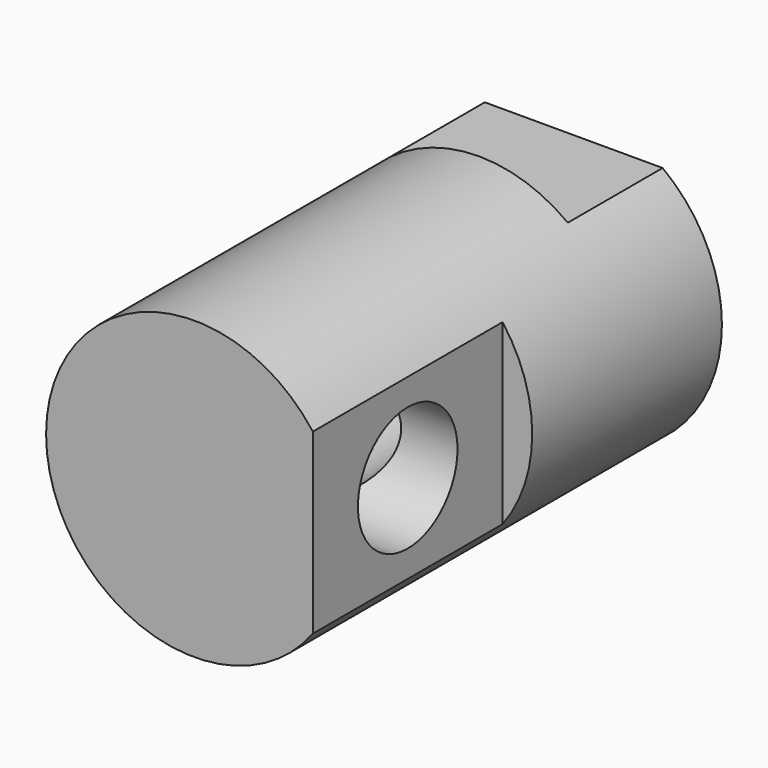
from build123d import *

# Parameters (mm, degrees)
F0_R     = 5
F1_DEPTH = 16
F2_W     = 4
F2_H     = 4.6315791518
F2_W_2   = 11.2692320682
F2_H_2   = 9.1250005215
F3_DEPTH = 12.5
F4_W     = 7.7142857378
F4_H     = 14.8317284754
F5_DEPTH = 12.5
F6_R     = 2.1
F7_DEPTH = 12.5
F8_R     = 2.1
F9_DEPTH = 12


# Not quite as in the source:
# - a feature names something its author has since deleted; it is built from what else it names


with BuildPart() as f1:
    # F0 (on Front) → F1 (new body)
    with BuildSketch(Plane.XZ):
        Circle(F0_R)
    extrude(amount=F1_DEPTH)

    # F2 (on Right) → F3 (cut, symmetric)
    with BuildSketch(Plane.YZ):
        with Locations((-2, 6.3157895759)):
            Rectangle(F2_W, F2_H)
        with Locations((1.6346160341, -8.5625002608)):
            Rectangle(F2_W_2, F2_H_2)
    extrude(amount=F3_DEPTH, both=True, mode=Mode.SUBTRACT)

    # F4 (on Top) → F5 (cut, symmetric)
    with BuildSketch(Plane.XY):
        with Locations((7.8571428689, -15.4158642377)):
            Rectangle(F4_W, F4_H)
    extrude(amount=F5_DEPTH, both=True, mode=Mode.SUBTRACT)

    # F6 (on Right) → F7 (cut, symmetric)
    with BuildSketch(Plane.YZ):
        with Locations((-12, 0)):
            Circle(F6_R)
    extrude(amount=F7_DEPTH, both=True, mode=Mode.SUBTRACT)

    # F8 (on Front) → F9 (cut)
    with BuildSketch(Plane.XZ):
        Circle(F8_R)
    extrude(amount=F9_DEPTH, mode=Mode.SUBTRACT)


solid = f1.part
